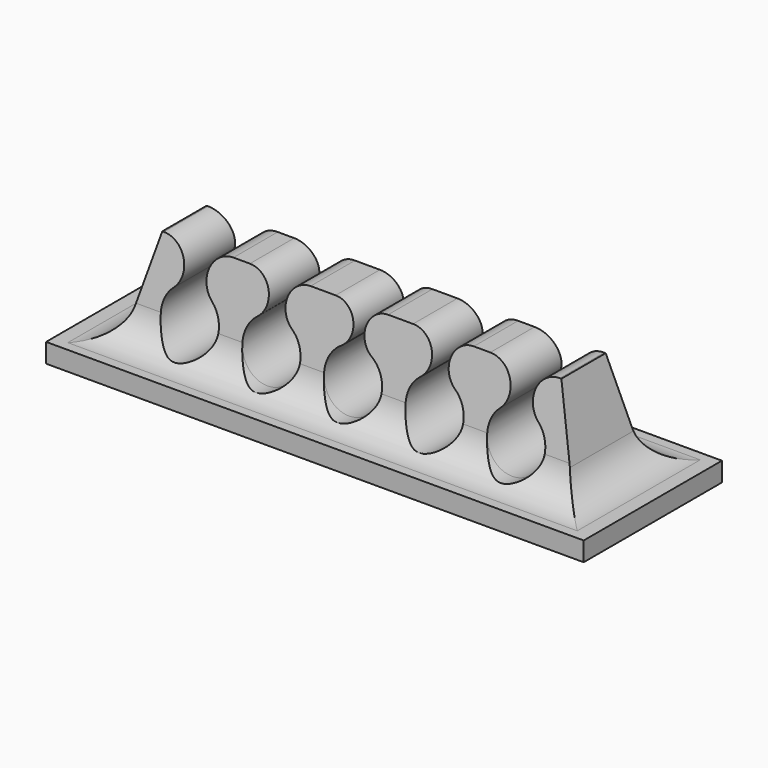
from build123d import *

# Parameters (mm, degrees)
F1_DEPTH      = 12.7
F3_DEPTH      = 30.481
F3_DEPTH_BACK = 30.481
F4_W          = 71.12
F4_H          = 22.86
F4_W_2        = 60.96
F4_H_2        = 12.7
F5_DEPTH      = 2.54
F6_T4_DEPTH   = 80.9119487344
F6_S6_R       = 3.81
F6_T7_DEPTH   = 42
F6_S8_R       = 3.81
F6_T9_DEPTH   = 42
F6_S10_R      = 3.81
F6_T11_DEPTH  = 42
F6_S12_R      = 3.81
F6_T13_DEPTH  = 42
F6_S14_R      = 3.81
F6_T15_DEPTH  = 42
F6_T20_DEPTH  = 31.2943644327
F6_T26_DEPTH  = 80.9119487344
F6_S27_R      = 3.81
F6_T28_DEPTH  = 42
F6_S29_R      = 3.81
F6_T30_DEPTH  = 42
F6_S31_R      = 3.81
F6_T32_DEPTH  = 42
F6_S33_R      = 3.81
F6_T34_DEPTH  = 42
F6_S35_R      = 3.81
F6_T36_DEPTH  = 42
F6_T42_DEPTH  = 31.2943644327
F6_T49_DEPTH  = 80.9119487344
F6_T54_DEPTH  = 31.2943644327
F6_T62_DEPTH  = 80.9119487344
F6_T67_DEPTH  = 31.2943644327
F6_T75_DEPTH  = 80.9119487344
F6_T80_DEPTH  = 31.2943644327
F6_T88_DEPTH  = 80.9119487344
F6_T93_DEPTH  = 31.2943644327


# Not quite as in the source:
# - a fillet or chamfer that OpenCascade refuses, or shapes differently, is made with other operations: its cross-section is extruded or revolved along the edge and cut away or added


with BuildPart() as f1:
    # F0 (on Front) → F1 (new body)
    with BuildSketch(Plane.XZ):
        with BuildLine():
            Line((-26.3964543073, 15.24), (-30.48, 0))
            Line((-30.48, 0), (30.48, 0))
            Line((30.48, 0), (26.3964543073, 15.24))
            Line((26.3964543073, 15.24), (26.1890573268, 15.24))
            ThreePointArc((26.1890573268, 15.24), (23.2932552373, 13.2447934662), (24.1261503873, 9.8282448388))
            ThreePointArc((24.1261503873, 9.8282448388), (21.59, 3.175), (19.0538496127, 9.8282448388))
            ThreePointArc((19.0538496127, 9.8282448388), (19.8867447627, 13.2447934662), (16.9909426732, 15.24))
            Line((16.9909426732, 15.24), (14.8108354471, 15.24))
            ThreePointArc((14.8108354471, 15.24), (12.0679506957, 13.2621337872), (13.0783470803, 10.034987887))
            ThreePointArc((13.0783470803, 10.034987887), (10.795, 3.175), (8.5116529197, 10.034987887))
            ThreePointArc((8.5116529197, 10.034987887), (9.5220493043, 13.2621337872), (6.7791645529, 15.24))
            Line((6.7791645529, 15.24), (3.4721075882, 15.24))
            ThreePointArc((3.4721075882, 15.24), (0.8561705504, 13.2707158547), (2.0251855519, 10.2121850707))
            ThreePointArc((2.0251855519, 10.2121850707), (0, 3.175), (-2.0251855519, 10.2121850707))
            ThreePointArc((-2.0251855519, 10.2121850707), (-0.8561705504, 13.2707158547), (-3.4721075882, 15.24))
            Line((-3.4721075882, 15.24), (-6.7791645529, 15.24))
            ThreePointArc((-6.7791645529, 15.24), (-9.5220493043, 13.2621337872), (-8.5116529197, 10.034987887))
            ThreePointArc((-8.5116529197, 10.034987887), (-10.795, 3.175), (-13.0783470803, 10.034987887))
            ThreePointArc((-13.0783470803, 10.034987887), (-12.0679506957, 13.2621337872), (-14.8108354471, 15.24))
            Line((-14.8108354471, 15.24), (-16.9909426732, 15.24))
            ThreePointArc((-16.9909426732, 15.24), (-19.8867447627, 13.2447934662), (-19.0538496127, 9.8282448388))
            ThreePointArc((-19.0538496127, 9.8282448388), (-21.59, 3.175), (-24.1261503873, 9.8282448388))
            ThreePointArc((-24.1261503873, 9.8282448388), (-23.2932552373, 13.2447934662), (-26.1890573268, 15.24))
            Line((-26.1890573268, 15.24), (-26.3964543073, 15.24))
        make_face()
    extrude(amount=F1_DEPTH)

    # F2 (on Right) → F3 (cut, two sides)
    with BuildSketch(Plane.YZ) as f3_sk:
        Polygon((-12.7, 15.24), (-12.7, 0), (-10.012776814, 15.24), align=None)
        Polygon((-2.687223186, 15.24), (0, 0), (0, 15.24), align=None)
    extrude(amount=-F3_DEPTH, mode=Mode.SUBTRACT)
    extrude(f3_sk.sketch, amount=F3_DEPTH_BACK, mode=Mode.SUBTRACT)

    # F4 (on face) → F5 (join)
    with BuildSketch(Plane(origin=(0, 0, 0), x_dir=(1, 0, 0), z_dir=(0, 0, -1))):
        with Locations((0, 6.35)):
            Rectangle(F4_W, F4_H)
        with Locations((0, 6.35)):
            Rectangle(F4_W_2, F4_H_2, mode=Mode.SUBTRACT)
        with Locations((0, 6.35)):
            Rectangle(F4_W_2, F4_H_2)
    extrude(amount=-F5_DEPTH)

    # F6: fillet of radius 5.08 on 4 edges, made by hand


with BuildPart() as f6_tool2:
    # F6_s3 → F6_t4 (new body)
    with BuildSketch(Plane.YZ.offset(40.4559743672)):
        with BuildLine():
            ThreePointArc((-11.5119322101, 6.7378672575), (-13.2493945382, 3.728494229), (-16.5147555954, 2.54))
            Line((-16.5147555954, 2.54), (-12.252129469, 2.54))
            Line((-12.252129469, 2.54), (-11.5119322101, 6.7378672575))
        make_face()
    extrude(amount=-F6_T4_DEPTH)

    split(bisect_by=Plane(origin=(28.4382271537, 0, 7.62), x_dir=(0, 1, 0), z_dir=(-0.9659258263, 0, -0.2588190451)), keep=Keep.TOP)

    # F6_s6 → F6_t7 (cut, symmetric)
    with BuildSketch(Plane.XZ.offset(14)):
        with Locations((21.59, 6.985)):
            Circle(F6_S6_R)
    extrude(amount=F6_T7_DEPTH, both=True, mode=Mode.SUBTRACT)

    # F6_s8 → F6_t9 (cut, symmetric)
    with BuildSketch(Plane.XZ.offset(14)):
        with Locations((10.795, 6.985)):
            Circle(F6_S8_R)
    extrude(amount=F6_T9_DEPTH, both=True, mode=Mode.SUBTRACT)

    # F6_s10 → F6_t11 (cut, symmetric)
    with BuildSketch(Plane.XZ.offset(14)):
        with Locations((0, 6.985)):
            Circle(F6_S10_R)
    extrude(amount=F6_T11_DEPTH, both=True, mode=Mode.SUBTRACT)

    # F6_s12 → F6_t13 (cut, symmetric)
    with BuildSketch(Plane.XZ.offset(14)):
        with Locations((-10.795, 6.985)):
            Circle(F6_S12_R)
    extrude(amount=F6_T13_DEPTH, both=True, mode=Mode.SUBTRACT)

    # F6_s14 → F6_t15 (cut, symmetric)
    with BuildSketch(Plane.XZ.offset(14)):
        with Locations((-21.59, 6.985)):
            Circle(F6_S14_R)
    extrude(amount=F6_T15_DEPTH, both=True, mode=Mode.SUBTRACT)

    split(bisect_by=Plane(origin=(-28.4382271537, 0, 7.62), x_dir=(0, 1, 0), z_dir=(0.9659258263, 0, -0.2588190451)), keep=Keep.TOP)


with BuildPart() as f1_1:
    add(f1.part)

    # F6_t1: union F6_tool2
    add(f6_tool2.part)


with BuildPart() as f6_tool18:
    # F6_s19 → F6_t20 (new body)
    with BuildSketch(Plane.XZ.offset(21.9971822163)):
        with BuildLine():
            ThreePointArc((-33.6974301502, 2.54), (-30.6049220908, 3.5897650313), (-28.7905269526, 6.3051992509))
            Line((-28.7905269526, 6.3051992509), (-29.7994090512, 2.54))
            Line((-29.7994090512, 2.54), (-33.6974301502, 2.54))
        make_face()
    extrude(amount=-F6_T20_DEPTH)

    split(bisect_by=Plane(origin=(0, 0, 0), x_dir=(1, 0, 0), z_dir=(0, -0.984807753, -0.1736481777)), keep=Keep.TOP)

    split(bisect_by=Plane(origin=(0, -12.317048142, 2.1718279101), x_dir=(1, 0, 0), z_dir=(0, 0.984807753, -0.1736481777)), keep=Keep.TOP)


with BuildPart() as f1_2:
    add(f1_1.part)

    # F6_t17: union F6_tool18
    add(f6_tool18.part)


with BuildPart() as f6_tool24:
    # F6_s25 → F6_t26 (new body)
    with BuildSketch(Plane.YZ.offset(-40.4559743672)):
        with BuildLine():
            ThreePointArc((-1.1880677899, 6.7378672575), (0.5493945382, 3.728494229), (3.8147555954, 2.54))
            Line((3.8147555954, 2.54), (-0.447870531, 2.54))
            Line((-0.447870531, 2.54), (-1.1880677899, 6.7378672575))
        make_face()
    extrude(amount=F6_T26_DEPTH)

    # F6_s27 → F6_t28 (cut, symmetric)
    with BuildSketch(Plane.XZ.offset(-1.3)):
        with Locations((-21.59, 6.985)):
            Circle(F6_S27_R)
    extrude(amount=F6_T28_DEPTH, both=True, mode=Mode.SUBTRACT)

    # F6_s29 → F6_t30 (cut, symmetric)
    with BuildSketch(Plane.XZ.offset(-1.3)):
        with Locations((-10.795, 6.985)):
            Circle(F6_S29_R)
    extrude(amount=F6_T30_DEPTH, both=True, mode=Mode.SUBTRACT)

    # F6_s31 → F6_t32 (cut, symmetric)
    with BuildSketch(Plane.XZ.offset(-1.3)):
        with Locations((0, 6.985)):
            Circle(F6_S31_R)
    extrude(amount=F6_T32_DEPTH, both=True, mode=Mode.SUBTRACT)

    # F6_s33 → F6_t34 (cut, symmetric)
    with BuildSketch(Plane.XZ.offset(-1.3)):
        with Locations((10.795, 6.985)):
            Circle(F6_S33_R)
    extrude(amount=F6_T34_DEPTH, both=True, mode=Mode.SUBTRACT)

    # F6_s35 → F6_t36 (cut, symmetric)
    with BuildSketch(Plane.XZ.offset(-1.3)):
        with Locations((21.59, 6.985)):
            Circle(F6_S35_R)
    extrude(amount=F6_T36_DEPTH, both=True, mode=Mode.SUBTRACT)

    split(bisect_by=Plane(origin=(28.4382271537, 0, 7.62), x_dir=(0, 1, 0), z_dir=(-0.9659258263, 0, -0.2588190451)), keep=Keep.TOP)

    split(bisect_by=Plane(origin=(-28.4382271537, 0, 7.62), x_dir=(0, 1, 0), z_dir=(0.9659258263, 0, -0.2588190451)), keep=Keep.TOP)


with BuildPart() as f1_3:
    add(f1_2.part)

    # F6_t23: union F6_tool24
    add(f6_tool24.part)


with BuildPart() as f6_tool40:
    # F6_s41 → F6_t42 (new body)
    with BuildSketch(Plane.XZ.offset(-9.2971822163)):
        with BuildLine():
            ThreePointArc((28.7905269526, 6.3051992509), (30.6049220908, 3.5897650313), (33.6974301502, 2.54))
            Line((33.6974301502, 2.54), (29.7994090512, 2.54))
            Line((29.7994090512, 2.54), (28.7905269526, 6.3051992509))
        make_face()
    extrude(amount=F6_T42_DEPTH)

    split(bisect_by=Plane(origin=(0, 0, 0), x_dir=(1, 0, 0), z_dir=(0, -0.984807753, -0.1736481777)), keep=Keep.TOP)

    split(bisect_by=Plane(origin=(0, -12.317048142, 2.1718279101), x_dir=(1, 0, 0), z_dir=(0, 0.984807753, -0.1736481777)), keep=Keep.TOP)


with BuildPart() as f1_4:
    add(f1_3.part)

    # F6_t39: union F6_tool40
    add(f6_tool40.part)


with BuildPart() as f6_tool47:
    # F6_s48 → F6_t49 (new body)
    with BuildSketch(Plane.YZ.offset(40.4559743672)):
        with BuildLine():
            ThreePointArc((-11.5119322101, 6.7378672575), (-13.2493945382, 3.728494229), (-16.5147555954, 2.54))
            Line((-16.5147555954, 2.54), (-12.252129469, 2.54))
            Line((-12.252129469, 2.54), (-11.5119322101, 6.7378672575))
        make_face()
    extrude(amount=-F6_T49_DEPTH)

    split(bisect_by=Plane(origin=(28.4382271537, 0, 7.62), x_dir=(0, 1, 0), z_dir=(0.9659258263, 0, 0.2588190451)), keep=Keep.TOP)

    split(bisect_by=Plane.YZ.offset(35.56), keep=Keep.BOTTOM)


with BuildPart() as f6_tool52:
    # F6_s53 → F6_t54 (new body)
    with BuildSketch(Plane.XZ.offset(-9.2971822163)):
        with BuildLine():
            ThreePointArc((28.7905269526, 6.3051992509), (30.6049220908, 3.5897650313), (33.6974301502, 2.54))
            Line((33.6974301502, 2.54), (29.7994090512, 2.54))
            Line((29.7994090512, 2.54), (28.7905269526, 6.3051992509))
        make_face()
    extrude(amount=F6_T54_DEPTH)

    split(bisect_by=Plane(origin=(0, -12.317048142, 2.1718279101), x_dir=(1, 0, 0), z_dir=(0, -0.984807753, 0.1736481777)), keep=Keep.TOP)

    split(bisect_by=Plane.XZ.offset(17.78), keep=Keep.BOTTOM)


with BuildPart() as f6_tool47_1:
    add(f6_tool47.part)

    # F6_t57: intersect F6_tool52
    add(f6_tool52.part, mode=Mode.INTERSECT)


with BuildPart() as f1_5:
    add(f1_4.part)

    # F6_t45: union F6_tool47
    add(f6_tool47_1.part)


with BuildPart() as f6_tool60:
    # F6_s61 → F6_t62 (new body)
    with BuildSketch(Plane.YZ.offset(40.4559743672)):
        with BuildLine():
            ThreePointArc((-11.5119322101, 6.7378672575), (-13.2493945382, 3.728494229), (-16.5147555954, 2.54))
            Line((-16.5147555954, 2.54), (-12.252129469, 2.54))
            Line((-12.252129469, 2.54), (-11.5119322101, 6.7378672575))
        make_face()
    extrude(amount=-F6_T62_DEPTH)

    split(bisect_by=Plane(origin=(-28.4382271537, 0, 7.62), x_dir=(0, 1, 0), z_dir=(-0.9659258263, 0, 0.2588190451)), keep=Keep.TOP)

    split(bisect_by=Plane.YZ.offset(-35.56), keep=Keep.TOP)


with BuildPart() as f6_tool65:
    # F6_s66 → F6_t67 (new body)
    with BuildSketch(Plane.XZ.offset(21.9971822163)):
        with BuildLine():
            ThreePointArc((-33.6974301502, 2.54), (-30.6049220908, 3.5897650313), (-28.7905269526, 6.3051992509))
            Line((-28.7905269526, 6.3051992509), (-29.7994090512, 2.54))
            Line((-29.7994090512, 2.54), (-33.6974301502, 2.54))
        make_face()
    extrude(amount=-F6_T67_DEPTH)

    split(bisect_by=Plane(origin=(0, -12.317048142, 2.1718279101), x_dir=(1, 0, 0), z_dir=(0, -0.984807753, 0.1736481777)), keep=Keep.TOP)

    split(bisect_by=Plane.XZ.offset(17.78), keep=Keep.BOTTOM)


with BuildPart() as f6_tool60_1:
    add(f6_tool60.part)

    # F6_t70: intersect F6_tool65
    add(f6_tool65.part, mode=Mode.INTERSECT)


with BuildPart() as f1_6:
    add(f1_5.part)

    # F6_t58: union F6_tool60
    add(f6_tool60_1.part)


with BuildPart() as f6_tool73:
    # F6_s74 → F6_t75 (new body)
    with BuildSketch(Plane.YZ.offset(-40.4559743672)):
        with BuildLine():
            ThreePointArc((-1.1880677899, 6.7378672575), (0.5493945382, 3.728494229), (3.8147555954, 2.54))
            Line((3.8147555954, 2.54), (-0.447870531, 2.54))
            Line((-0.447870531, 2.54), (-1.1880677899, 6.7378672575))
        make_face()
    extrude(amount=F6_T75_DEPTH)

    split(bisect_by=Plane(origin=(-28.4382271537, 0, 7.62), x_dir=(0, 1, 0), z_dir=(-0.9659258263, 0, 0.2588190451)), keep=Keep.TOP)

    split(bisect_by=Plane.YZ.offset(-35.56), keep=Keep.TOP)


with BuildPart() as f6_tool78:
    # F6_s79 → F6_t80 (new body)
    with BuildSketch(Plane.XZ.offset(21.9971822163)):
        with BuildLine():
            ThreePointArc((-33.6974301502, 2.54), (-30.6049220908, 3.5897650313), (-28.7905269526, 6.3051992509))
            Line((-28.7905269526, 6.3051992509), (-29.7994090512, 2.54))
            Line((-29.7994090512, 2.54), (-33.6974301502, 2.54))
        make_face()
    extrude(amount=-F6_T80_DEPTH)

    split(bisect_by=Plane(origin=(0, 0, 0), x_dir=(1, 0, 0), z_dir=(0, 0.984807753, 0.1736481777)), keep=Keep.TOP)

    split(bisect_by=Plane.XZ.offset(-5.08), keep=Keep.TOP)


with BuildPart() as f6_tool73_1:
    add(f6_tool73.part)

    # F6_t83: intersect F6_tool78
    add(f6_tool78.part, mode=Mode.INTERSECT)


with BuildPart() as f1_7:
    add(f1_6.part)

    # F6_t71: union F6_tool73
    add(f6_tool73_1.part)


with BuildPart() as f6_tool86:
    # F6_s87 → F6_t88 (new body)
    with BuildSketch(Plane.YZ.offset(-40.4559743672)):
        with BuildLine():
            ThreePointArc((-1.1880677899, 6.7378672575), (0.5493945382, 3.728494229), (3.8147555954, 2.54))
            Line((3.8147555954, 2.54), (-0.447870531, 2.54))
            Line((-0.447870531, 2.54), (-1.1880677899, 6.7378672575))
        make_face()
    extrude(amount=F6_T88_DEPTH)

    split(bisect_by=Plane(origin=(28.4382271537, 0, 7.62), x_dir=(0, 1, 0), z_dir=(0.9659258263, 0, 0.2588190451)), keep=Keep.TOP)

    split(bisect_by=Plane.YZ.offset(35.56), keep=Keep.BOTTOM)


with BuildPart() as f6_tool91:
    # F6_s92 → F6_t93 (new body)
    with BuildSketch(Plane.XZ.offset(-9.2971822163)):
        with BuildLine():
            ThreePointArc((28.7905269526, 6.3051992509), (30.6049220908, 3.5897650313), (33.6974301502, 2.54))
            Line((33.6974301502, 2.54), (29.7994090512, 2.54))
            Line((29.7994090512, 2.54), (28.7905269526, 6.3051992509))
        make_face()
    extrude(amount=F6_T93_DEPTH)

    split(bisect_by=Plane(origin=(0, 0, 0), x_dir=(1, 0, 0), z_dir=(0, 0.984807753, 0.1736481777)), keep=Keep.TOP)

    split(bisect_by=Plane.XZ.offset(-5.08), keep=Keep.TOP)


with BuildPart() as f6_tool86_1:
    add(f6_tool86.part)

    # F6_t96: intersect F6_tool91
    add(f6_tool91.part, mode=Mode.INTERSECT)


with BuildPart() as f1_8:
    add(f1_7.part)

    # F6_t84: union F6_tool86
    add(f6_tool86_1.part)


solid = f1_8.part
